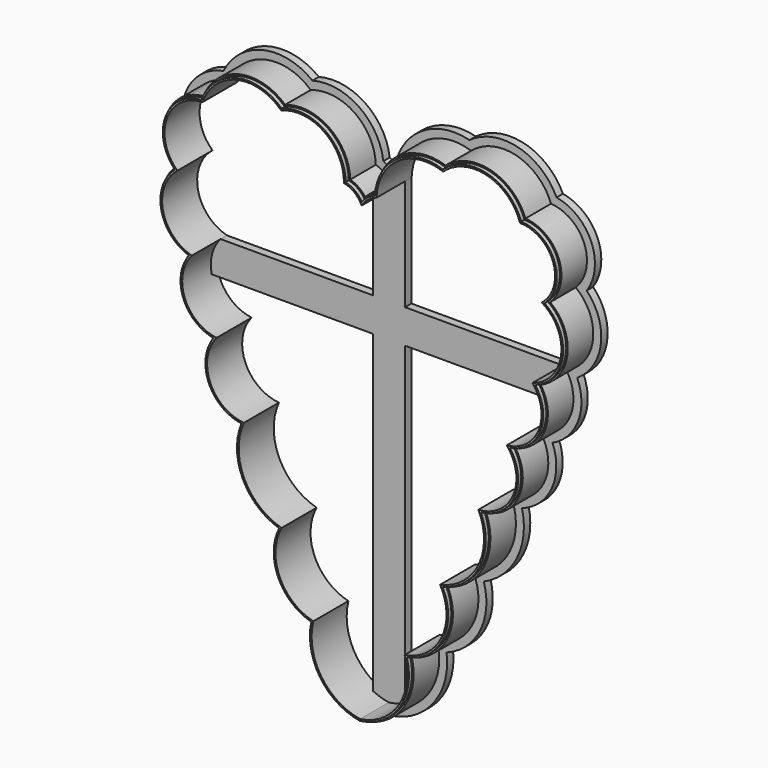
from build123d import *

# Parameters (mm, degrees)
F1_DEPTH = 11
F3_DEPTH = 10
F5_DEPTH = 2
F6_W     = 8
F6_H     = 8.5
F7_DEPTH = 2


with BuildPart() as f1:
    # F0 (on Front) → F1 (new body)
    with BuildSketch(Plane.XZ):
        with BuildLine():
            ThreePointArc((39.0705500579, -8.52496936), (46.72096884, -2.3164746642), (45.4314010117, 7.451397609))
            ThreePointArc((45.4314010117, 7.451397609), (52.3349438106, 16.1264631775), (47.7886465249, 26.2381814678))
            ThreePointArc((47.7886465249, 26.2381814678), (50.2701969547, 36.2833369913), (41.9150114031, 42.3869520205))
            ThreePointArc((41.9150114031, 42.3869520205), (33.4367867693, 50.2079291964), (22.2244569704, 47.5002295437))
            ThreePointArc((22.2244569704, 47.5002295437), (10.8566281912, 46.1253851638), (5.2163100926, 36.1602188347))
            ThreePointArc((5.2163100926, 36.1602188347), (3.3871782253, 35.1886396049), (1.9242797709, 33.7224821441))
            ThreePointArc((1.9242797709, 33.7224821441), (0.2060931662, 35.6601876437), (-2.1423101686, 36.7519154435))
            ThreePointArc((-2.1423101686, 36.7519154435), (-7.2708907681, 46.4831703255), (-18.1895864419, 47.8179906611))
            ThreePointArc((-18.1895864419, 47.8179906611), (-29.5124145758, 50.8897432152), (-38.3332962899, 43.1544897295))
            ThreePointArc((-38.3332962899, 43.1544897295), (-47.3249375206, 36.5242237511), (-44.9588955164, 25.6058042591))
            ThreePointArc((-44.9588955164, 25.6058042591), (-48.3852347219, 15.6615137302), (-41.4218344822, 7.7786353488))
            ThreePointArc((-41.4218344822, 7.7786353488), (-42.8868566438, -2.0549157562), (-35.2681064262, -8.4423770976))
            ThreePointArc((-35.2681064262, -8.4423770976), (-36.4780330886, -18.7288037829), (-28.2643223371, -25.0382769915))
            ThreePointArc((-28.2643223371, -25.0382769915), (-27.9422707168, -37.1366223637), (-18.8030679193, -45.0706409052))
            ThreePointArc((-18.8030679193, -45.0706409052), (-19.0455768915, -56.0125901141), (-10.7319048048, -63.1307302875))
            ThreePointArc((-10.7319048048, -63.1307302875), (-8.5024893952, -74.7301167227), (1.486939211, -81.0330822839))
            ThreePointArc((1.486939211, -81.0330822839), (11.4330463974, -74.7729616567), (13.2165865743, -63.1568890473))
            ThreePointArc((13.2165865743, -63.1568890473), (22.3038978548, -56.1642100409), (22.1972204462, -44.6983735723))
            ThreePointArc((22.1972204462, -44.6983735723), (31.5494835172, -37.1283643345), (31.8068847226, -25.0990830165))
            ThreePointArc((31.8068847226, -25.0990830165), (40.2572033461, -18.9237451092), (39.0705500579, -8.52496936))
        make_face()
        with BuildLine():
            ThreePointArc((-18.287823031, 47.3288657516), (-7.4780325298, 46.1157556728), (-2.5663635332, 36.4101534549))
            ThreePointArc((-2.5663635332, 36.4101534549), (0.1022138006, 35.2102271012), (1.8737317574, 32.8815252377))
            ThreePointArc((1.8737317574, 32.8815252377), (3.4685951698, 34.7220338469), (5.6255866592, 35.8527190194))
            ThreePointArc((5.6255866592, 35.8527190194), (11.074771804, 45.7660203722), (22.3176378772, 47.0170698967))
            ThreePointArc((22.3176378772, 47.0170698967), (33.3495644247, 49.796633279), (41.6101485742, 41.9740937007))
            ThreePointArc((41.6101485742, 41.9740937007), (49.9194357762, 36.0161229225), (47.0874105005, 26.1915973646))
            ThreePointArc((47.0874105005, 26.1915973646), (51.915995427, 16.1612135783), (44.7295889669, 7.6594847256))
            ThreePointArc((44.7295889669, 7.6594847256), (46.3044950278, -2.2263904431), (38.2778021949, -8.2082847183))
            ThreePointArc((38.2778021949, -8.2082847183), (39.8992064768, -18.6937143429), (31.1706150566, -24.7257022472))
            ThreePointArc((31.1706150566, -24.7257022472), (31.1846152182, -36.91843323), (21.5669627376, -44.4126740578))
            ThreePointArc((21.5669627376, -44.4126740578), (21.9428314543, -55.9461967568), (12.6780636079, -62.8256952773))
            ThreePointArc((12.6780636079, -62.8256952773), (11.2241235412, -74.3211876976), (1.491255675, -80.6086013792))
            ThreePointArc((1.491255675, -80.6086013792), (-8.2859760991, -74.2989428398), (-10.2277903072, -62.8256952773))
            ThreePointArc((-10.2277903072, -62.8256952773), (-18.6823826488, -55.7956537612), (-18.1915944439, -44.8110853891))
            ThreePointArc((-18.1915944439, -44.8110853891), (-27.5735039539, -36.9338984851), (-27.6541622004, -24.6838456762))
            ThreePointArc((-27.6541622004, -24.6838456762), (-36.1203277284, -18.4954623496), (-34.4911439915, -8.1360315111))
            ThreePointArc((-34.4911439915, -8.1360315111), (-42.4788506232, -1.9460435419), (-40.6942105462, 8.0005371815))
            ThreePointArc((-40.6942105462, 8.0005371815), (-47.9577840613, 15.6667852228), (-44.3252140818, 25.5832006329))
            ThreePointArc((-44.3252140818, 25.5832006329), (-46.9652913596, 36.2864155083), (-38.0336352662, 42.7481750312))
            ThreePointArc((-38.0336352662, 42.7481750312), (-29.4229096781, 50.4793548119), (-18.287823031, 47.3288657516))
        make_face(mode=Mode.SUBTRACT)
    extrude(amount=F1_DEPTH)

    # F2 (on Front) → F3 (join)
    with BuildSketch(Plane.XZ):
        with BuildLine():
            ThreePointArc((-28.7894182833, -25.3380623372), (-28.2780674719, -37.315411053), (-19.3336110619, -45.2975825271))
            ThreePointArc((-19.3336110619, -45.2975825271), (-19.3757403856, -56.2049968971), (-11.1765373084, -63.3985031367))
            ThreePointArc((-11.1765373084, -63.3985031367), (-8.6987912382, -75.1140963115), (1.4829988261, -81.416913151))
            ThreePointArc((1.4829988261, -81.416913151), (11.6228084753, -75.1730955299), (13.6873525382, -63.445407948))
            ThreePointArc((13.6873525382, -63.445407948), (22.6321998986, -56.3579224617), (22.740727836, -44.9460441542))
            ThreePointArc((22.740727836, -44.9460441542), (31.8823212597, -37.3126706934), (32.3495800111, -25.4123013725))
            ThreePointArc((32.3495800111, -25.4123013725), (40.5882309676, -19.1148961819), (39.7155861385, -8.781882453))
            ThreePointArc((39.7155861385, -8.781882453), (47.09182758, -2.4119959763), (46.0226495696, 7.2751733683))
            ThreePointArc((46.0226495696, 7.2751733683), (52.7137277602, 16.0930995605), (48.3826353269, 26.279756913))
            ThreePointArc((48.3826353269, 26.279756913), (50.5908388805, 36.5118212888), (42.1872958021, 42.7529564461))
            ThreePointArc((42.1872958021, 42.7529564461), (33.5173854794, 50.579592633), (22.1412690395, 47.9324141817))
            ThreePointArc((22.1412690395, 47.9324141817), (10.6568550393, 46.4488985081), (4.851078209, 36.4296400985))
            ThreePointArc((4.851078209, 36.4296400985), (3.2803936817, 35.5805678874), (1.9607699749, 34.377834843))
            ThreePointArc((1.9607699749, 34.377834843), (0.3310806886, 36.0394522047), (-1.766727365, 37.0474506157))
            ThreePointArc((-1.766727365, 37.0474506157), (-7.079102033, 46.8124644401), (-18.1016485533, 48.254784727))
            ThreePointArc((-18.1016485533, 48.254784727), (-29.594023844, 51.2608992563), (-38.6011454354, 43.5160186875))
            ThreePointArc((-38.6011454354, 43.5160186875), (-47.6524591085, 36.7317470687), (-45.5066577228, 25.6255255231))
            ThreePointArc((-45.5066577228, 25.6255255231), (-48.7691918651, 15.6449376796), (-42.0299203098, 7.5927031056))
            ThreePointArc((-42.0299203098, 7.5927031056), (-43.2526434444, -2.1619201779), (-35.9042109813, -8.6924842885))
            ThreePointArc((-35.9042109813, -8.6924842885), (-36.8086632261, -18.922394093), (-28.7894182833, -25.3380623372))
        make_face()
        with BuildLine():
            ThreePointArc((1.491255675, -80.6086013792), (-8.2859760991, -74.2989428398), (-10.2277903072, -62.8256952773))
            ThreePointArc((-10.2277903072, -62.8256952773), (-18.6823826488, -55.7956537612), (-18.1915944439, -44.8110853891))
            ThreePointArc((-18.1915944439, -44.8110853891), (-27.5735039539, -36.9338984851), (-27.6541622004, -24.6838456762))
            ThreePointArc((-27.6541622004, -24.6838456762), (-36.1203277284, -18.4954623496), (-34.4911439915, -8.1360315111))
            ThreePointArc((-34.4911439915, -8.1360315111), (-42.4788506232, -1.9460435419), (-40.6942105462, 8.0005371815))
            ThreePointArc((-40.6942105462, 8.0005371815), (-47.9577840613, 15.6667852228), (-44.3252140818, 25.5832006329))
            ThreePointArc((-44.3252140818, 25.5832006329), (-46.9652913596, 36.2864155083), (-38.0336352662, 42.7481750312))
            ThreePointArc((-38.0336352662, 42.7481750312), (-29.4229096781, 50.4793548119), (-18.287823031, 47.3288657516))
            ThreePointArc((-18.287823031, 47.3288657516), (-7.4780325298, 46.1157556728), (-2.5663635332, 36.4101534549))
            ThreePointArc((-2.5663635332, 36.4101534549), (0.1022138006, 35.2102271012), (1.8737317574, 32.8815252377))
            ThreePointArc((1.8737317574, 32.8815252377), (3.4685951698, 34.7220338469), (5.6255866592, 35.8527190194))
            ThreePointArc((5.6255866592, 35.8527190194), (11.074771804, 45.7660203722), (22.3176378772, 47.0170698967))
            ThreePointArc((22.3176378772, 47.0170698967), (33.3495644247, 49.796633279), (41.6101485742, 41.9740937007))
            ThreePointArc((41.6101485742, 41.9740937007), (49.9194357762, 36.0161229225), (47.0874105005, 26.1915973646))
            ThreePointArc((47.0874105005, 26.1915973646), (51.915995427, 16.1612135783), (44.7295889669, 7.6594847256))
            ThreePointArc((44.7295889669, 7.6594847256), (46.3044950278, -2.2263904431), (38.2778021949, -8.2082847183))
            ThreePointArc((38.2778021949, -8.2082847183), (39.8992064768, -18.6937143429), (31.1706150566, -24.7257022472))
            ThreePointArc((31.1706150566, -24.7257022472), (31.1846152182, -36.91843323), (21.5669627376, -44.4126740578))
            ThreePointArc((21.5669627376, -44.4126740578), (21.9428314543, -55.9461967568), (12.6780636079, -62.8256952773))
            ThreePointArc((12.6780636079, -62.8256952773), (11.2241235412, -74.3211876976), (1.491255675, -80.6086013792))
        make_face(mode=Mode.SUBTRACT)
    extrude(amount=F3_DEPTH)

    # F4 (on Front) → F5 (join)
    with BuildSketch(Plane.XZ):
        with BuildLine():
            ThreePointArc((-31.2933360918, -26.7145614825), (-30.0626590432, -38.2196991357), (-21.8890280635, -46.4096023724))
            ThreePointArc((-21.8890280635, -46.4096023724), (-21.1276893783, -57.1828959351), (-13.3885235772, -64.716076106))
            ThreePointArc((-13.3885235772, -64.716076106), (-9.7350068872, -77.0674278864), (1.4618042214, -83.434177136))
            ThreePointArc((1.4618042214, -83.434177136), (12.6270411685, -77.1886920415), (15.9893100479, -64.845120916))
            ThreePointArc((15.9893100479, -64.845120916), (24.3740160314, -57.347499456), (25.3313999659, -46.140312566))
            ThreePointArc((25.3313999659, -46.140312566), (33.6545641024, -38.2407900675), (34.9013631871, -26.8336427909))
            ThreePointArc((34.9013631871, -26.8336427909), (42.3740651436, -20.0204664993), (42.5637323356, -9.9098447543))
            ThreePointArc((42.5637323356, -9.9098447543), (49.009962504, -2.9964088065), (48.7536090239, 6.4525997595))
            ThreePointArc((48.7536090239, 6.4525997595), (54.7055223286, 15.9043679712), (51.1515112452, 26.4935227786))
            ThreePointArc((51.1515112452, 26.4935227786), (52.3061738341, 37.6104413128), (43.5808496442, 44.5952706717))
            ThreePointArc((43.5808496442, 44.5952706717), (33.9591097891, 52.5310125566), (21.7167574574, 50.1480130832))
            ThreePointArc((21.7167574574, 50.1480130832), (9.581408462, 48.1355293439), (2.9826864127, 37.7541203183))
            ThreePointArc((2.9826864127, 37.7541203183), (2.5321333274, 37.4861496239), (2.0973058773, 37.1933502652))
            ThreePointArc((2.0973058773, 37.1933502652), (1.1564435593, 37.8965061856), (0.1297728303, 38.4671175807))
            ThreePointArc((0.1297728303, 38.4671175807), (-6.0288252744, 48.5169345665), (-17.6498973059, 50.4861569773))
            ThreePointArc((-17.6498973059, 50.4861569773), (-30.0301798203, 53.2128100125), (-39.9733990154, 45.3490689213))
            ThreePointArc((-39.9733990154, 45.3490689213), (-49.3958373956, 37.7573118999), (-48.1412388738, 25.7222339089))
            ThreePointArc((-48.1412388738, 25.7222339089), (-50.7716397612, 15.4759489819), (-44.8075162442, 6.7389818703))
            ThreePointArc((-44.8075162442, 6.7389818703), (-45.158666704, -2.7743885235), (-38.7333983934, -9.798877831))
            ThreePointArc((-38.7333983934, -9.798877831), (-38.5942671383, -19.8317147245), (-31.2933360918, -26.7145614825))
        make_face()
        with BuildLine():
            ThreePointArc((1.491255675, -80.6086013792), (-8.2859760991, -74.2989428398), (-10.2277903072, -62.8256952773))
            ThreePointArc((-10.2277903072, -62.8256952773), (-18.6823826488, -55.7956537612), (-18.1915944439, -44.8110853891))
            ThreePointArc((-18.1915944439, -44.8110853891), (-27.5735039539, -36.9338984851), (-27.6541622004, -24.6838456762))
            ThreePointArc((-27.6541622004, -24.6838456762), (-36.1203277284, -18.4954623496), (-34.4911439915, -8.1360315111))
            ThreePointArc((-34.4911439915, -8.1360315111), (-42.4788506232, -1.9460435419), (-40.6942105462, 8.0005371815))
            ThreePointArc((-40.6942105462, 8.0005371815), (-47.9577840613, 15.6667852228), (-44.3252140818, 25.5832006329))
            ThreePointArc((-44.3252140818, 25.5832006329), (-46.9652913596, 36.2864155083), (-38.0336352662, 42.7481750312))
            ThreePointArc((-38.0336352662, 42.7481750312), (-29.4229096781, 50.4793548119), (-18.287823031, 47.3288657516))
            ThreePointArc((-18.287823031, 47.3288657516), (-7.4780325298, 46.1157556728), (-2.5663635332, 36.4101534549))
            ThreePointArc((-2.5663635332, 36.4101534549), (0.1022138006, 35.2102271012), (1.8737317574, 32.8815252377))
            ThreePointArc((1.8737317574, 32.8815252377), (3.4685951698, 34.7220338469), (5.6255866592, 35.8527190194))
            ThreePointArc((5.6255866592, 35.8527190194), (11.074771804, 45.7660203722), (22.3176378772, 47.0170698967))
            ThreePointArc((22.3176378772, 47.0170698967), (33.3495644247, 49.796633279), (41.6101485742, 41.9740937007))
            ThreePointArc((41.6101485742, 41.9740937007), (49.9194357762, 36.0161229225), (47.0874105005, 26.1915973646))
            ThreePointArc((47.0874105005, 26.1915973646), (51.915995427, 16.1612135783), (44.7295889669, 7.6594847256))
            ThreePointArc((44.7295889669, 7.6594847256), (46.3044950278, -2.2263904431), (38.2778021949, -8.2082847183))
            ThreePointArc((38.2778021949, -8.2082847183), (39.8992064768, -18.6937143429), (31.1706150566, -24.7257022472))
            ThreePointArc((31.1706150566, -24.7257022472), (31.1846152182, -36.91843323), (21.5669627376, -44.4126740578))
            ThreePointArc((21.5669627376, -44.4126740578), (21.9428314543, -55.9461967568), (12.6780636079, -62.8256952773))
            ThreePointArc((12.6780636079, -62.8256952773), (11.2241235412, -74.3211876976), (1.491255675, -80.6086013792))
        make_face(mode=Mode.SUBTRACT)
    extrude(amount=F5_DEPTH)

    # F6 (on Front) → F7 (join)
    with BuildSketch(Plane.XZ):
        Polygon((-2.4262682426, 8.0005371815), (-42.5083744706, 8.0005371815), (-43.8785292208, -0.4994628185), (-2.4262682426, -0.4994628185), align=None)
        Polygon((-2.4262682426, 36.4266432116), (-2.4262682426, 8.0005371815), (5.5737317574, 8.0005371815), (5.5737317574, 35.8574517777), (2.2378848509, 35.5696513543), align=None)
        with Locations((1.5737317574, 3.7505371815)):
            Rectangle(F6_W, F6_H)
        Polygon((5.5737317574, -0.4994628185), (-2.4262682426, -0.4994628185), (-2.4262682426, -80.5981069097), (0.7191397591, -81.807880033), (5.5737317574, -80.5055871606), align=None)
        Polygon((47.3726280034, 8.0005371815), (5.5737317574, 8.0005371815), (5.5737317574, -0.4994628185), (48.0919629335, -0.4994628185), align=None)
    extrude(amount=F7_DEPTH)


solid = f1.part
